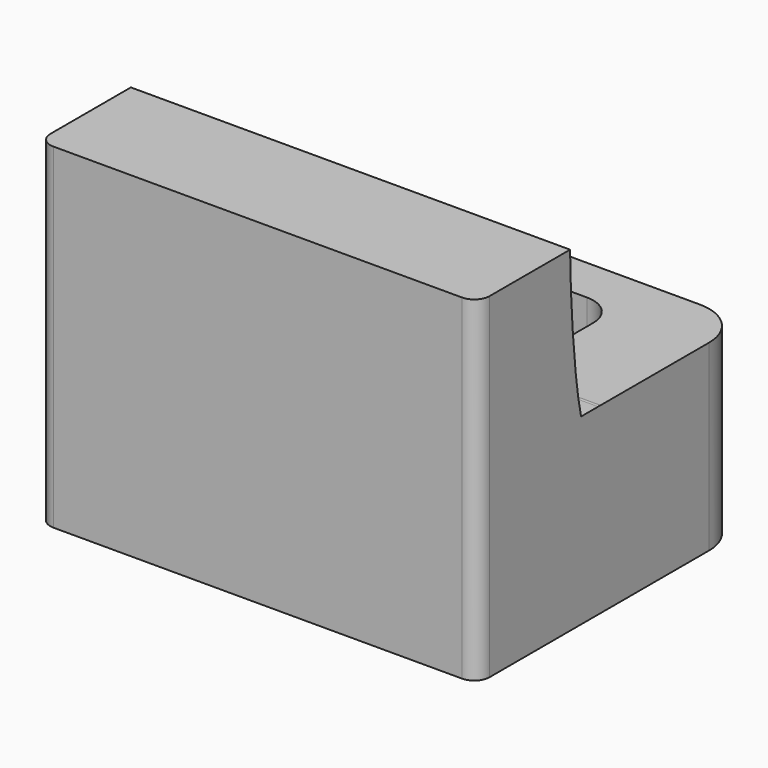
from build123d import *

# Parameters (mm, degrees)
F1_DEPTH = 6
F3_DEPTH = 4
F5_DEPTH = 5
F6_W     = 13
F6_H     = 3.4
F7_DEPTH = 10
F9_DEPTH = 14.4


# Not quite as in the source:
# - a feature names something its author has since deleted; it is built from what else it names


with BuildPart() as f1:
    # F0 (on Top) → F1 (new body)
    with BuildSketch(Plane.XY):
        with BuildLine():
            ThreePointArc((0, 3.3761399509), (0.1464466094, 3.0225865603), (0.5, 2.8761399509))
            Line((0.5, 2.8761399509), (13.9, 2.8761399509))
            ThreePointArc((13.9, 2.8761399509), (14.2535533906, 3.0225865603), (14.4, 3.3761399509))
            Line((14.4, 3.3761399509), (0, 3.3761399509))
        make_face()
        with BuildLine():
            Line((0, 12.3761399509), (0, 3.3761399509))
            Line((0, 3.3761399509), (14.4, 3.3761399509))
            Line((14.4, 3.3761399509), (14.4, 12.3761399509))
            ThreePointArc((14.4, 12.3761399509), (13.9606601718, 13.4368001227), (12.9, 13.8761399509))
            Line((12.9, 13.8761399509), (1.5, 13.8761399509))
            ThreePointArc((1.5, 13.8761399509), (0.4393398282, 13.4368001227), (0, 12.3761399509))
        make_face()
        with BuildLine():
            ThreePointArc((3, 11.3761399509), (3.2928932188, 12.0832467321), (4, 12.3761399509))
            Line((4, 12.3761399509), (10.4, 12.3761399509))
            ThreePointArc((10.4, 12.3761399509), (11.1071067812, 12.0832467321), (11.4, 11.3761399509))
            Line((11.4, 11.3761399509), (11.4, 10.5761399509))
            ThreePointArc((11.4, 10.5761399509), (11.1071067812, 9.8690331698), (10.4, 9.5761399509))
            Line((10.4, 9.5761399509), (4, 9.5761399509))
            ThreePointArc((4, 9.5761399509), (3.2928932188, 9.8690331698), (3, 10.5761399509))
            Line((3, 10.5761399509), (3, 11.3761399509))
        make_face(mode=Mode.SUBTRACT)
    extrude(amount=F1_DEPTH)

    # F2 (on Top) → F3 (cut)
    with BuildSketch(Plane.XY):
        with BuildLine():
            ThreePointArc((13.9, 11.8761399509), (13.4606601718, 12.9368001227), (12.4, 13.3761399509))
            Line((12.4, 13.3761399509), (2, 13.3761399509))
            ThreePointArc((2, 13.3761399509), (0.9393398282, 12.9368001227), (0.5, 11.8761399509))
            Line((0.5, 11.8761399509), (0.5, 4.8761399509))
            ThreePointArc((0.5, 4.8761399509), (0.9393398282, 3.8154797792), (2, 3.3761399509))
            Line((2, 3.3761399509), (12.4, 3.3761399509))
            ThreePointArc((12.4, 3.3761399509), (13.4606601718, 3.8154797792), (13.9, 4.8761399509))
            Line((13.9, 4.8761399509), (13.9, 11.8761399509))
        make_face()
    extrude(amount=F3_DEPTH, mode=Mode.SUBTRACT)

    # F4 (on face) → F5 (join)
    with BuildSketch(Plane.XY.offset(6)):
        with BuildLine():
            Line((14.4, 6.6761399509), (0, 6.6761399509))
            Line((0, 6.6761399509), (0, 3.3761399509))
            ThreePointArc((0, 3.3761399509), (0.1464466094, 3.0225865603), (0.5, 2.8761399509))
            Line((0.5, 2.8761399509), (13.9, 2.8761399509))
            ThreePointArc((13.9, 2.8761399509), (14.2535533906, 3.0225865603), (14.4, 3.3761399509))
            Line((14.4, 3.3761399509), (14.4, 6.6761399509))
        make_face()
    extrude(amount=F5_DEPTH)

    # F6 (on face) → F7 (cut)
    with BuildSketch(Plane(origin=(0, 0, 0), x_dir=(1, 0, 0), z_dir=(0, 0, -1))):
        with Locations((7.2, -4.7761399509)):
            Rectangle(F6_W, F6_H)
    extrude(amount=-F7_DEPTH, mode=Mode.SUBTRACT)

    # F8 (on Right) → F9 (join)
    with BuildSketch(Plane.YZ):
        with BuildLine():
            add(Edge.make_bspline(
                [(7.1272827151, 6), (6.8833303011, 6.9959140901), (6.6957208529, 9.2354907336), (6.6761399509, 11)],
                knots=[0.4613630388, 0.4613630388, 0.4613630388, 0.4613630388, 1, 1, 1, 1], degree=3))
            Line((6.6761399509, 11), (6.6761399509, 6))
            Line((6.6761399509, 6), (7.1272827151, 6))
        make_face()
        with BuildLine():
            add(Edge.make_bspline(
                [(7.9261399509, 6), (7.8912804031, 6.0110682928), (7.8586101723, 6.0100642713), (7.8278293535, 6)],
                knots=[0, 0, 0, 0, 0.0376755281, 0.0376755281, 0.0376755281, 0.0376755281], degree=3))
            Line((7.8278293535, 6), (7.9261399509, 6))
        make_face()
        with BuildLine():
            Line((7.8278293535, 6), (7.1272827151, 6))
            add(Edge.make_bspline(
                [(7.8278293535, 6), (7.6417958125, 5.9391734168), (7.4240615582, 5.2101966849), (7.2160450595, 5.6376356026), (7.1272827151, 6)],
                knots=[0.0376755281, 0.0376755281, 0.0376755281, 0.0376755281, 0.2653794095, 0.4613630388, 0.4613630388, 0.4613630388, 0.4613630388], degree=3))
        make_face()
    extrude(amount=F9_DEPTH)


solid = f1.part
